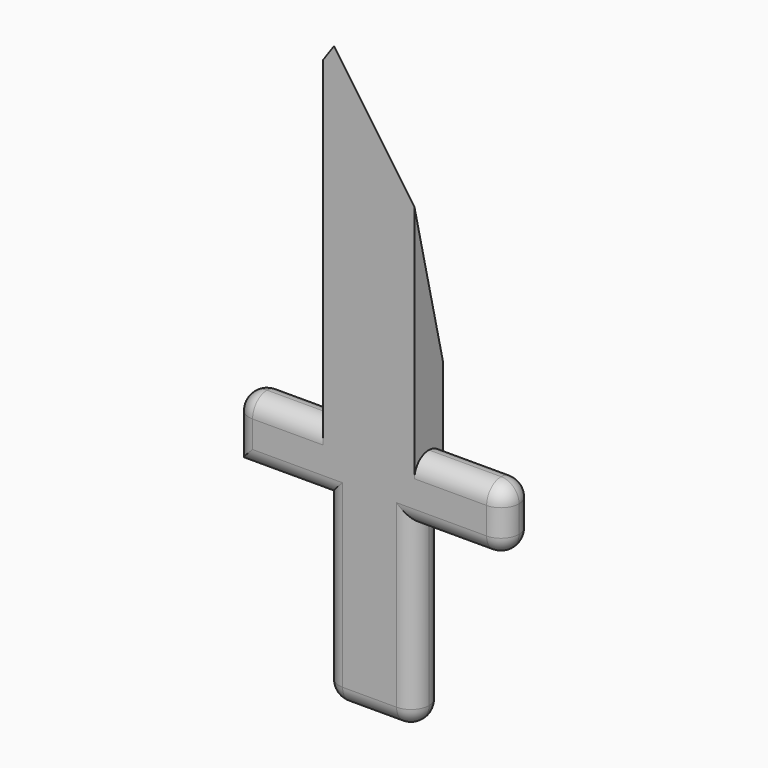
from build123d import *

# Parameters (mm, degrees)
F0_W        = 12.7
F0_H        = 8.8700183392
F0_H_2      = 25.4
F2_DEPTH    = 2.54
F3_DEPTH    = 2.54
F4_R        = 2.53999
F5_T1_DEPTH = 76.5737284666
F6_T1_DEPTH = 62.0182579324


# Not quite as in the source:
# - a fillet or chamfer that OpenCascade refuses, or shapes differently, is made with other operations: its cross-section is extruded or revolved along the edge and cut away or added
# - a fillet or chamfer is up to 0.001 mm smaller than in the source, because OpenCascade refuses the exact size


with BuildPart() as f2:
    # F0 (on Front) → F2 (new body, symmetric)
    with BuildSketch(Plane.XZ):
        with Locations((-23.8077666163, 5.7760581046)):
            Rectangle(F0_W, F0_H)
        with Locations((-23.8077666163, -11.3589510649)):
            Rectangle(F0_W, F0_H_2)
        with Locations((-36.5077666163, 5.7760581046)):
            Rectangle(F0_W, F0_H)
        with Locations((-11.1077666163, 5.7760581046)):
            Rectangle(F0_W, F0_H)
    extrude(amount=F2_DEPTH, both=True)

    # F1 (on Front) → F3 (join, symmetric)
    with BuildSketch(Plane.XZ):
        Polygon((-30.3534455597, 10.2110672742), (-17.4847040325, 10.2110672742), (-17.4847040325, 55.5314160883), (-23.9190747961, 64.7633413825), (-30.3534455597, 55.5314160883), align=None)
    extrude(amount=F3_DEPTH, both=True)

    # F4 (radius 2.54 in the source; OpenCascade refuses exactly that, so slightly less here)
    f4_edges = [f2.edges().sort_by_distance(p)[0] for p in [
        (-11.107767, 2.54, 1.341049),
        (-11.107767, -2.54, 1.341049),
        (-11.121235, 2.54, 10.211067),
        (-11.121235, -2.54, 10.211067),
        (-4.757767, -2.54, 5.776058),
        (-4.757767, 2.54, 5.776058),
        (-4.757767, 0, 10.211067),
        (-4.757767, 0, 1.341049),
        (-36.605606, -2.54, 10.211067),
        (-36.605606, 2.54, 10.211067),
        (-36.507767, -2.54, 1.341049),
        (-36.507767, 2.54, 1.341049),
        (-42.857767, -2.54, 5.776058),
        (-42.857767, 2.54, 5.776058),
        (-42.857767, 0, 10.211067),
        (-17.457767, 2.54, -11.358951),
        (-17.457767, -2.54, -11.358951),
        (-30.157767, -2.54, -11.358951),
        (-30.157767, 2.54, -11.358951),
        (-23.807767, -2.54, -24.058951),
        (-30.157767, 0, -24.058951),
        (-23.807767, 2.54, -24.058951),
        (-17.457767, 0, -24.058951),
    ]]
    fillet(f4_edges, radius=F4_R)

    # F5: chamfer of 12.7 on 1 edges, made by hand

    # F5_s2 → F5_t1 (cut)
    with BuildSketch(Plane(origin=(-13.0912626788, 0, 18.7831201367), x_dir=(0, 1, 0), z_dir=(-0.5717925773, 0, 0.8203982256))):
        Polygon((2.54, -4.7080313623), (-10.16, -17.4080313623), (2.54, -17.4080313623), align=None)
    extrude(amount=F5_T1_DEPTH, mode=Mode.SUBTRACT)

    # F6: chamfer of 7.62 on 1 edges, made by hand

    # F6_s2 → F6_t1 (cut)
    with BuildSketch(Plane(origin=(-10.0507456007, 0, 14.4206381549), x_dir=(0, 1, 0), z_dir=(-0.5717925773, 0, 0.8203982256))):
        Polygon((-2.8481536726, -10.0961850349), (2.54, 2.9119686377), (2.54, -4.7080313623), align=None)
    extrude(amount=F6_T1_DEPTH, mode=Mode.SUBTRACT)


solid = f2.part
